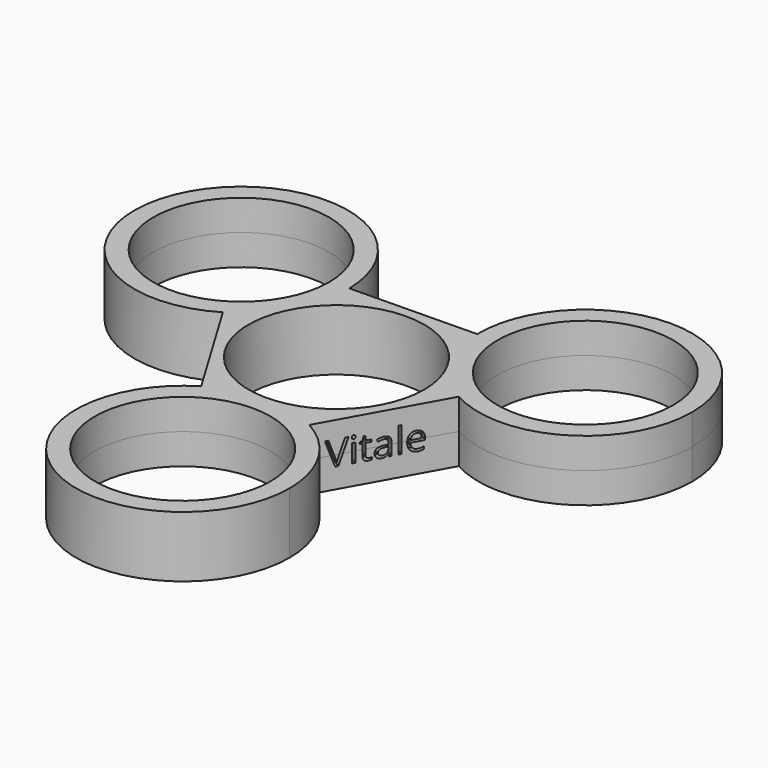
from build123d import *

# Parameters (mm, degrees)
F2_DEPTH     = 4
F0_R         = 11.5
F3_DEPTH     = 4
F4_TEXT_SIZE = 4.3920863795
F5_DEPTH     = 1
F6_TEXT_SIZE = 4.2948239651
F7_DEPTH     = 1


# Not quite as in the source:
# - Text() gives the source's letters only with a copy of the font that has no kerning and outlines rounded to 1/6400 em; it was checked with that copy


with BuildPart() as f2:
    # F1 (on Top) → F2 (new body, symmetric)
    with BuildSketch(Plane.XY):
        with BuildLine():
            ThreePointArc((-15.244216168, 0.490111409), (-10.2725191442, 5.5866107561), (-8.4582, 12.4714))
            ThreePointArc((-8.4582, 12.4714), (-8.4586469613, 12.5831492728), (-8.4599878167, 12.6948913949))
            Line((-8.4599878167, 12.6948913949), (-22.4282, 12.4714))
            Line((-22.4282, 12.4714), (-15.244216168, 0.490111409))
        make_face()
        with BuildLine():
            ThreePointArc((-8.4599878167, 12.6948913949), (-8.4586469613, 12.5831492728), (-8.4582, 12.4714))
            ThreePointArc((-8.4582, 12.4714), (-10.2725191442, 5.5866107561), (-15.244216168, 0.490111409))
            Line((-15.244216168, 0.490111409), (-6.752183832, -13.672711409))
            ThreePointArc((-6.752183832, -13.672711409), (0.2030555642, -11.6858728534), (7.2196216311, -13.4439067365))
            Line((7.2196216311, -13.4439067365), (15.2339783689, 0.9725067365))
            ThreePointArc((15.2339783689, 0.9725067365), (10.0375231751, 6.0036022298), (8.0535878167, 12.9591086051))
            Line((8.0535878167, 12.9591086051), (-8.4599878167, 12.6948913949))
        make_face()
        with BuildLine():
            Line((-22.4282, 12.4714), (-8.4599878167, 12.6948913949))
            ThreePointArc((-8.4599878167, 12.6948913949), (-34.6385649697, 19.2587328566), (-15.244216168, 0.490111409))
            Line((-15.244216168, 0.490111409), (-22.4282, 12.4714))
        make_face()
        with BuildLine():
            Line((22.0218, 13.1826), (8.0535878167, 12.9591086051))
            ThreePointArc((8.0535878167, 12.9591086051), (10.0375231751, 6.0036022298), (15.2339783689, 0.9725067365))
            Line((15.2339783689, 0.9725067365), (22.0218, 13.1826))
        make_face()
        with BuildLine():
            ThreePointArc((35.9918, 13.1826), (21.9100507272, 27.1521530387), (8.0535878167, 12.9591086051))
            Line((8.0535878167, 12.9591086051), (22.0218, 13.1826))
            Line((22.0218, 13.1826), (15.2339783689, 0.9725067365))
            ThreePointArc((15.2339783689, 0.9725067365), (29.1047030705, 1.1412801349), (35.9918, 13.1826))
        make_face()
        with BuildLine():
            Line((0.4318, -25.654), (-6.752183832, -13.672711409))
            ThreePointArc((-6.752183832, -13.672711409), (-6.4529892439, -37.8096808558), (14.4018, -25.654))
            ThreePointArc((14.4018, -25.654), (12.4731198651, -18.5710969295), (7.2196216311, -13.4439067365))
            Line((7.2196216311, -13.4439067365), (0.4318, -25.654))
        make_face()
        with BuildLine():
            ThreePointArc((7.2196216311, -13.4439067365), (0.2030555642, -11.6858728534), (-6.752183832, -13.672711409))
            Line((-6.752183832, -13.672711409), (0.4318, -25.654))
            Line((0.4318, -25.654), (7.2196216311, -13.4439067365))
        make_face()
    extrude(amount=F2_DEPTH, both=True)

    # F0 (on Top) → F3 (cut, symmetric)
    with BuildSketch(Plane.XY):
        with Locations((0.4195799751, -25.6597892816)):
            Circle(F0_R)
        with Locations((-22.4318193612, 12.4665277234)):
            Circle(F0_R)
        with Locations((22.0122393861, 13.1932615582)):
            Circle(F0_R)
        Circle(F0_R)
    extrude(amount=F3_DEPTH, both=True, mode=Mode.SUBTRACT)

    # F4 (on face) → F5 (cut)
    with BuildSketch(Plane(origin=(11.2244683987, -6.2398941392, 0), x_dir=(0.4858855856, 0.874022424, 0), z_dir=(0.874022424, -0.4858855856, 0))):
        with Locations((-6.5265540034, -1.3646098087)):
            Text('Vitale', F4_TEXT_SIZE, font='Open Sans', text_align=(TextAlign.LEFT, TextAlign.BOTTOM))
    extrude(amount=-F5_DEPTH, mode=Mode.SUBTRACT)

    # F6 (on face) → F7 (cut)
    with BuildSketch(Plane(origin=(-10.9967782473, -6.5936711676, 0), x_dir=(0.514243653, -0.8576441368, 0), z_dir=(-0.8576441368, -0.514243653, 0))):
        with Locations((-5.5817719549, -2.0431217272)):
            Text('2017', F6_TEXT_SIZE, font='Arimo', font_style=FontStyle.BOLD, text_align=(TextAlign.LEFT, TextAlign.BOTTOM))
    extrude(amount=-F7_DEPTH, mode=Mode.SUBTRACT)


solid = f2.part
